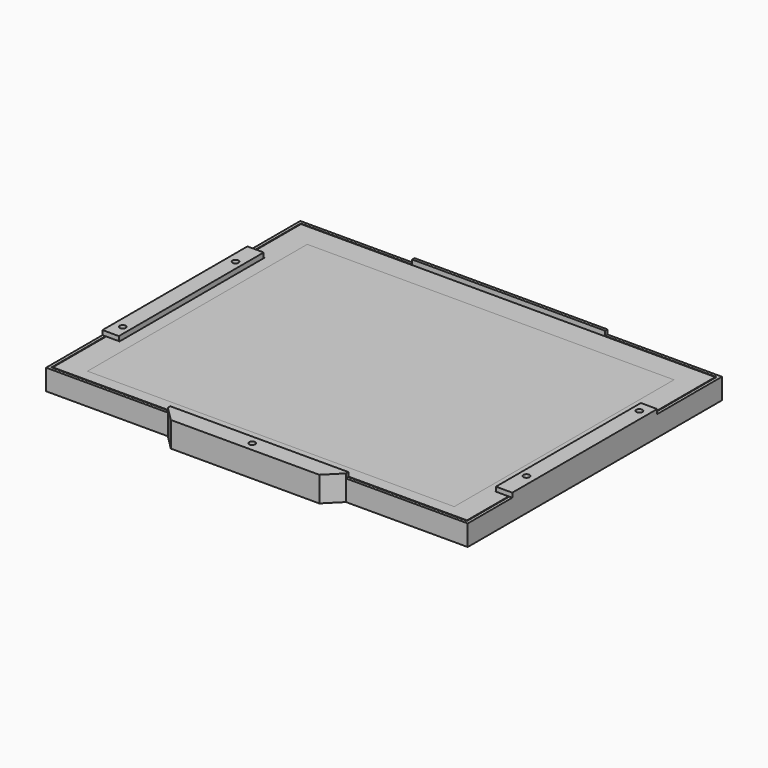
from build123d import *

# Parameters (mm, degrees)
F0_W      = 279
F0_H      = 209
F0_W_2    = 247
F0_H_2    = 185
F1_DEPTH  = 9
F2_W      = 9
F2_H      = 122
F3_DEPTH  = 25
F6_DEPTH  = 14
F7_W      = 280
F7_H      = 210
F8_DEPTH  = 5
F9_W      = 280
F9_H      = 145
F10_DEPTH = 2.9
F11_W     = 235
F11_H     = 69
F12_DEPTH = 25
F13_R     = 1.2
F14_DEPTH = 25
F15_W     = 11
F15_H     = 122
F15_W_2   = 130
F15_H_2   = 2
F16_DEPTH = 3
F17_R     = 2.05
F18_DEPTH = 25
F19_W     = 247
F19_H     = 185
F20_DEPTH = 2


with BuildPart() as f1:
    # F0 (on Top) → F1 (new body)
    with BuildSketch(Plane.XY):
        Rectangle(F0_W, F0_H)
        with Locations((1, -4)):
            Rectangle(F0_W_2, F0_H_2, mode=Mode.SUBTRACT)
    extrude(amount=F1_DEPTH)

    # F2 (on face) → F3 (cut)
    with BuildSketch(Plane.XY.offset(9)):
        with Locations((-135, 1.5)):
            Rectangle(F2_W, F2_H)
        with Locations((135, -8.5)):
            Rectangle(F2_W, F2_H)
    extrude(amount=-F3_DEPTH, mode=Mode.SUBTRACT)


with BuildPart() as f6:
    # F5 (on offset) → F6 (new body)
    with BuildSketch(Plane.XY.offset(-5)):
        Polygon((142, 107), (-142, 107), (-142, -107), (-60, -107), (60, -107), (142, -107), align=None)
        Polygon((-140, 62.5), (-140, 105), (140, 105), (140, 52.5), (131, 52.5), (131, -69.5), (140, -69.5), (140, -105), (-140, -105), (-140, -59.5), (-131, -59.5), (-131, 62.5), align=None, mode=Mode.SUBTRACT)
        Polygon((60, -107), (-60, -107), (-50, -117), (50, -117), align=None)
    extrude(amount=F6_DEPTH)

    # F7 (on face) → F8 (join)
    with BuildSketch(Plane(origin=(0, 0, -5), x_dir=(1, 0, 0), z_dir=(0, 0, -1))):
        Rectangle(F7_W, F7_H)
    extrude(amount=-F8_DEPTH)

    # F9 (on face) → F10 (join)
    with BuildSketch(Plane.XY):
        with Locations((0, -32.5)):
            Rectangle(F9_W, F9_H)
    extrude(amount=F10_DEPTH)

    # F11 (on face) → F12 (cut)
    with BuildSketch(Plane.XY.offset(2.9)):
        with Locations((0, 54)):
            Rectangle(F11_W, F11_H)
    extrude(amount=-F12_DEPTH, mode=Mode.SUBTRACT)

    # F13 (on face) → F14 (cut)
    with BuildSketch(Plane(origin=(0, 0, -5), x_dir=(1, 0, 0), z_dir=(0, 0, -1))):
        with Locations((90, -6.5)):
            Circle(F13_R)
        with Locations((90, 100.5)):
            Circle(F13_R)
        with Locations((60, 60.5)):
            Circle(F13_R)
        with Locations((60, -6.5)):
            Circle(F13_R)
        with Locations((-60, 60.5)):
            Circle(F13_R)
        with Locations((-60, -6.5)):
            Circle(F13_R)
    extrude(amount=-F14_DEPTH, mode=Mode.SUBTRACT)

    # F15 (on face) → F16 (join)
    with BuildSketch(Plane.XY.offset(9)):
        with Locations((-136.5, 1.5)):
            Rectangle(F15_W, F15_H)
        with Locations((136.5, -8.5)):
            Rectangle(F15_W, F15_H)
        with Locations((0, 106)):
            Rectangle(F15_W_2, F15_H_2)
        Polygon((-60, -107), (-50, -117), (50, -117), (60, -107), (60, -105), (-60, -105), align=None)
    extrude(amount=F16_DEPTH)

    # F17 (on face) → F18 (cut)
    with BuildSketch(Plane.XY.offset(12)):
        with Locations((-136, 45)):
            Circle(F17_R)
        with Locations((-136, -50)):
            Circle(F17_R)
        with Locations((136, -50)):
            Circle(F17_R)
        with Locations((136, 45)):
            Circle(F17_R)
        with Locations((0, -111)):
            Circle(F17_R)
    extrude(amount=-F18_DEPTH, mode=Mode.SUBTRACT)


with BuildPart() as f20:
    # F19 (on face) → F20 (new body)
    with BuildSketch(Plane.XY.offset(9)):
        with Locations((1, -4)):
            Rectangle(F19_W, F19_H)
    extrude(amount=-F20_DEPTH)


solid = Compound([f1.part, f6.part, f20.part])
